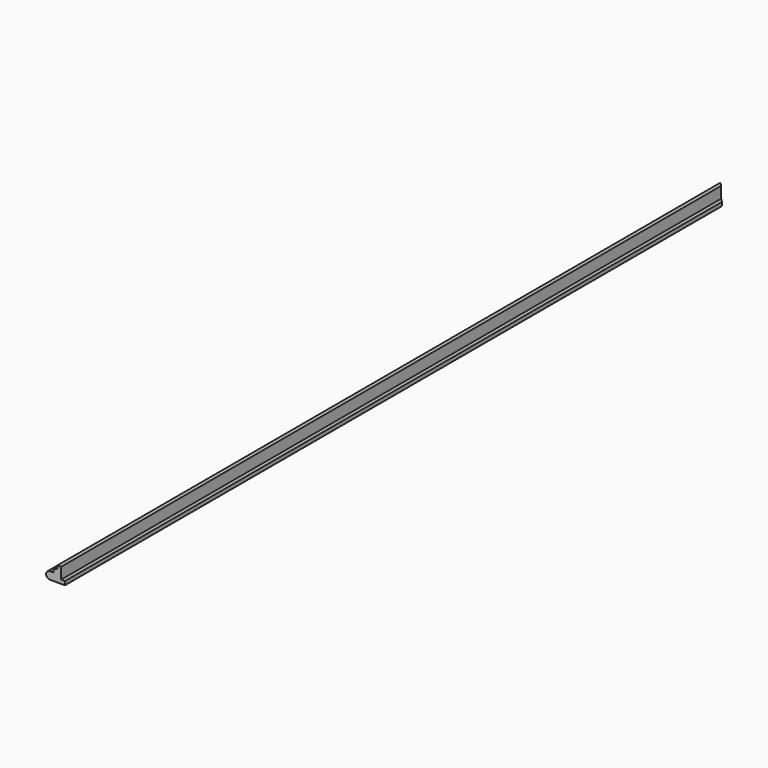
from build123d import *

# Parameters (mm, degrees)
F1_DEPTH = 1447.8
F2_R     = 3.17499
F3_R     = 6.34999
F5_DEPTH = 58.42


# Not quite as in the source:
# - a fillet or chamfer is up to 0.001 mm smaller than in the source, because OpenCascade refuses the exact size


with BuildPart() as f1:
    # F0 (on Front) → F1 (new body)
    with BuildSketch(Plane.XZ):
        Polygon((-6.35, 6.35), (-6.35, 25.4), (-12.7, 25.4), (-12.7, 19.05), (-19.05, 19.05), (-19.05, 12.7), (-31.75, 12.7), (-31.75, 0), (0, 0), (0, 6.35), align=None)
    extrude(amount=F1_DEPTH)

    # F2 (radius 3.175 in the source; OpenCascade refuses exactly that, so slightly less here)
    f2_edges = [f1.edges().sort_by_distance(p)[0] for p in [
        (-12.7, -723.9, 19.05),
        (-19.05, -723.9, 19.05),
    ]]
    fillet(f2_edges, radius=F2_R)

    # F3 (radius 6.35 in the source; OpenCascade refuses exactly that, so slightly less here)
    f3_edges = [f1.edges().sort_by_distance(p)[0] for p in [
        (-31.75, -723.9, 12.7),
        (-31.75, -723.9, 0),
    ]]
    fillet(f3_edges, radius=F3_R)

    # F4 (on face) → F5 (cut, symmetric)
    with BuildSketch(Plane.XY.offset(6.35)):
        Polygon((-49.2702007145, -18.9922992855), (0, -68.2625), (0, 0), (-49.2702007145, 0), align=None)
    extrude(amount=F5_DEPTH, both=True, mode=Mode.SUBTRACT)


solid = f1.part
